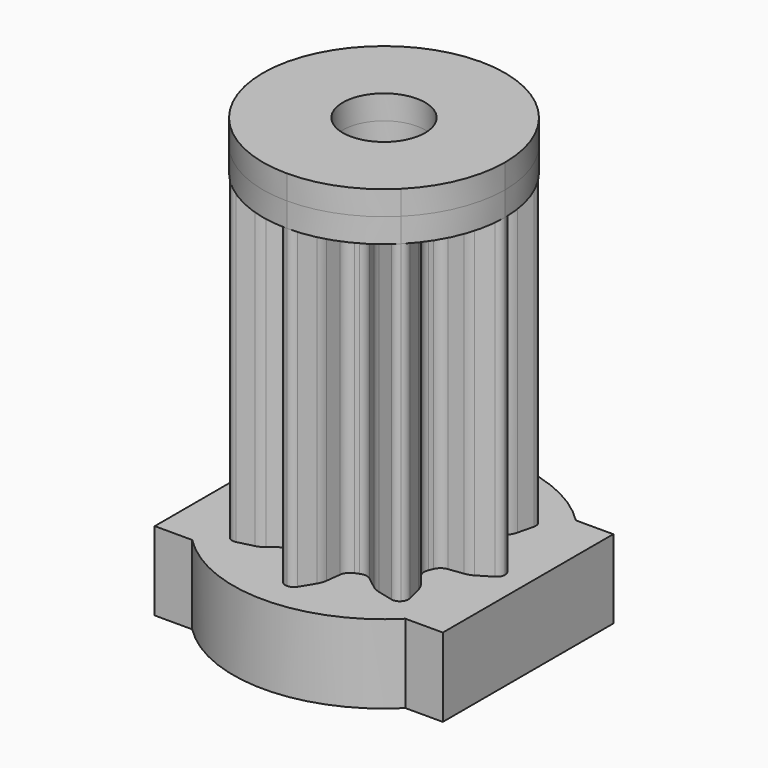
from build123d import *
from build123d import SkipClean  # not in build123d's __all__

# Parameters (mm, degrees)
F0_R     = 5
F0_R_2   = 3.15
F0_R_3   = 2.55
F1_DEPTH = 3.25
F2_R     = 2.55
F3_DEPTH = 14
F5_DEPTH = 1


# Not quite as in the source:
# - a feature names something its author has since deleted; it is built from what else it names


with BuildPart() as f1:
    # F0 (on Top) → F1 (new body)
    with BuildSketch(Plane.XY):
        with BuildLine():
            Line((-5.95, -4.4), (-4.4034787385, -4.4))
            ThreePointArc((-4.4034787385, -4.4), (0, -6.225), (4.4034787385, -4.4))
            Line((4.4034787385, -4.4), (5.95, -4.4))
            Line((5.95, -4.4), (5.95, 4.4))
            Line((5.95, 4.4), (4.4034787385, 4.4))
            ThreePointArc((4.4034787385, 4.4), (0, 6.225), (-4.4034787385, 4.4))
            Line((-4.4034787385, 4.4), (-5.95, 4.4))
            Line((-5.95, 4.4), (-5.95, -4.4))
        make_face()
        Circle(F0_R, mode=Mode.SUBTRACT)
        Circle(F0_R)
        Circle(F0_R_2, mode=Mode.SUBTRACT)
        Circle(F0_R_2)
        Circle(F0_R_3, mode=Mode.SUBTRACT)
        Circle(F0_R_3)
        with BuildLine():
            ThreePointArc((-1.275, -1.1244443072), (-0.601040764, 1.5902043894), (1.7, 0))
            ThreePointArc((1.7, 0), (1.5902043894, -0.601040764), (1.275, -1.1244443072))
            ThreePointArc((1.275, -1.1244443072), (0, -1.7), (-1.275, -1.1244443072))
        make_face(mode=Mode.SUBTRACT)
        with BuildLine():
            Line((1.275, -1.1244443072), (-1.275, -1.1244443072))
            ThreePointArc((-1.275, -1.1244443072), (0, -1.7), (1.275, -1.1244443072))
        make_face()
    extrude(amount=F1_DEPTH)

    # F2 (on face) → F3 (join)
    with BuildSketch(Plane.XY.offset(3.25)):
        with BuildLine():
            ThreePointArc((-4.8302633262, 0.3000085552), (-4.9546244936, 0.172348246), (-5, 0))
            ThreePointArc((-5, 0), (-4.9546244936, -0.172348246), (-4.8302633262, -0.3000085552))
            Line((-4.8302633262, -0.3000085552), (-4.2601369618, -0.6425750355))
            ThreePointArc((-4.2601369618, -0.6425750355), (-4.0929165173, -0.7205512094), (-3.9131380826, -0.7620563314))
            Line((-3.9131380826, -0.7620563314), (-3.3117988826, -0.835891501))
            ThreePointArc((-3.3117988826, -0.835891501), (-3.0868883315, -0.9291389359), (-2.9422567869, -1.125))
            ThreePointArc((-2.9422567869, -1.125), (-3.15, 0), (-2.9422567869, 1.125))
            ThreePointArc((-2.9422567869, 1.125), (-3.0868883315, 0.9291389359), (-3.3117988826, 0.835891501))
            Line((-3.3117988826, 0.835891501), (-3.9131380826, 0.7620563314))
            ThreePointArc((-3.9131380826, 0.7620563314), (-4.0929165173, 0.7205512094), (-4.2601369618, 0.6425750355))
            Line((-4.2601369618, 0.6425750355), (-4.8302633262, 0.3000085552))
        make_face()
        with BuildLine():
            ThreePointArc((-3.2033738691, 3.6276500367), (-3.3815799641, 3.6253171911), (-3.5355339059, 3.5355339059))
            ThreePointArc((-3.5355339059, 3.5355339059), (-3.6253171911, 3.3815799641), (-3.6276500367, 3.2033738691))
            Line((-3.6276500367, 3.2033738691), (-3.4667408995, 2.5580025694))
            ThreePointArc((-3.4667408995, 2.5580025694), (-3.4036356706, 2.3846223779), (-3.3058616735, 2.2281512744))
            Line((-3.3058616735, 2.2281512744), (-2.9328599965, 1.7507308991))
            ThreePointArc((-2.9328599965, 1.7507308991), (-2.8397601142, 1.5257592297), (-2.8759848548, 1.2849945972))
            ThreePointArc((-2.8759848548, 1.2849945972), (-2.2273863607, 2.2273863607), (-1.2849945972, 2.8759848548))
            ThreePointArc((-1.2849945972, 2.8759848548), (-1.5257592297, 2.8397601142), (-1.7507308991, 2.9328599965))
            Line((-1.7507308991, 2.9328599965), (-2.2281512744, 3.3058616735))
            ThreePointArc((-2.2281512744, 3.3058616735), (-2.3846223779, 3.4036356706), (-2.5580025694, 3.4667408995))
            Line((-2.5580025694, 3.4667408995), (-3.2033738691, 3.6276500367))
        make_face()
        with BuildLine():
            ThreePointArc((0.3000085552, 4.8302633262), (0.172348246, 4.9546244936), (0, 5))
            ThreePointArc((0, 5), (-0.172348246, 4.9546244936), (-0.3000085552, 4.8302633262))
            Line((-0.3000085552, 4.8302633262), (-0.6425750355, 4.2601369618))
            ThreePointArc((-0.6425750355, 4.2601369618), (-0.7205512094, 4.0929165173), (-0.7620563314, 3.9131380826))
            Line((-0.7620563314, 3.9131380826), (-0.835891501, 3.3117988826))
            ThreePointArc((-0.835891501, 3.3117988826), (-0.9291389359, 3.0868883315), (-1.125, 2.9422567869))
            ThreePointArc((-1.125, 2.9422567869), (0, 3.15), (1.125, 2.9422567869))
            ThreePointArc((1.125, 2.9422567869), (0.9291389359, 3.0868883315), (0.835891501, 3.3117988826))
            Line((0.835891501, 3.3117988826), (0.7620563314, 3.9131380826))
            ThreePointArc((0.7620563314, 3.9131380826), (0.7205512094, 4.0929165173), (0.6425750355, 4.2601369618))
            Line((0.6425750355, 4.2601369618), (0.3000085552, 4.8302633262))
        make_face()
        with BuildLine():
            ThreePointArc((3.2033738691, -3.6276500367), (3.3815799667, -3.6253171904), (3.5355339096, -3.5355339023))
            ThreePointArc((3.5355339096, -3.5355339023), (3.6253171918, -3.3815799616), (3.6276500367, -3.2033738691))
            Line((3.6276500367, -3.2033738691), (3.4667408995, -2.5580025694))
            ThreePointArc((3.4667408995, -2.5580025694), (3.4036356706, -2.3846223779), (3.3058616735, -2.2281512744))
            Line((3.3058616735, -2.2281512744), (2.9328599965, -1.7507308991))
            ThreePointArc((2.9328599965, -1.7507308991), (2.8397601142, -1.5257592297), (2.8759848548, -1.2849945972))
            ThreePointArc((2.8759848548, -1.2849945972), (2.2273863607, -2.2273863607), (1.2849945972, -2.8759848548))
            ThreePointArc((1.2849945972, -2.8759848548), (1.5257592297, -2.8397601142), (1.7507308991, -2.9328599965))
            Line((1.7507308991, -2.9328599965), (2.2281512744, -3.3058616735))
            ThreePointArc((2.2281512744, -3.3058616735), (2.3846223779, -3.4036356706), (2.5580025694, -3.4667408995))
            Line((2.5580025694, -3.4667408995), (3.2033738691, -3.6276500367))
        make_face()
        with BuildLine():
            ThreePointArc((-0.3000085552, -4.8302633262), (-0.172348246, -4.9546244936), (0, -5))
            ThreePointArc((0, -5), (0.172348246, -4.9546244936), (0.3000085552, -4.8302633262))
            Line((0.3000085552, -4.8302633262), (0.6425750355, -4.2601369618))
            ThreePointArc((0.6425750355, -4.2601369618), (0.7205512094, -4.0929165173), (0.7620563314, -3.9131380826))
            Line((0.7620563314, -3.9131380826), (0.835891501, -3.3117988826))
            ThreePointArc((0.835891501, -3.3117988826), (0.9291389359, -3.0868883315), (1.125, -2.9422567869))
            ThreePointArc((1.125, -2.9422567869), (0, -3.15), (-1.125, -2.9422567869))
            ThreePointArc((-1.125, -2.9422567869), (-0.9291389359, -3.0868883315), (-0.835891501, -3.3117988826))
            Line((-0.835891501, -3.3117988826), (-0.7620563314, -3.9131380826))
            ThreePointArc((-0.7620563314, -3.9131380826), (-0.7205512094, -4.0929165173), (-0.6425750355, -4.2601369618))
            Line((-0.6425750355, -4.2601369618), (-0.3000085552, -4.8302633262))
        make_face()
        with BuildLine():
            ThreePointArc((-3.6276500367, -3.2033738691), (-3.6253171911, -3.3815799641), (-3.5355339059, -3.5355339059))
            ThreePointArc((-3.5355339059, -3.5355339059), (-3.3815799641, -3.6253171911), (-3.2033738691, -3.6276500367))
            Line((-3.2033738691, -3.6276500367), (-2.5580025694, -3.4667408995))
            ThreePointArc((-2.5580025694, -3.4667408995), (-2.3846223779, -3.4036356706), (-2.2281512744, -3.3058616735))
            Line((-2.2281512744, -3.3058616735), (-1.7507308991, -2.9328599965))
            ThreePointArc((-1.7507308991, -2.9328599965), (-1.5257592297, -2.8397601142), (-1.2849945972, -2.8759848548))
            ThreePointArc((-1.2849945972, -2.8759848548), (-2.2273863607, -2.2273863607), (-2.8759848548, -1.2849945972))
            ThreePointArc((-2.8759848548, -1.2849945972), (-2.8397601142, -1.5257592297), (-2.9328599965, -1.7507308991))
            Line((-2.9328599965, -1.7507308991), (-3.3058616735, -2.2281512744))
            ThreePointArc((-3.3058616735, -2.2281512744), (-3.4036356706, -2.3846223779), (-3.4667408995, -2.5580025694))
            Line((-3.4667408995, -2.5580025694), (-3.6276500367, -3.2033738691))
        make_face()
        with BuildLine():
            ThreePointArc((2.8759848548, -1.2849945972), (2.9102205274, -1.205452812), (2.9422567869, -1.125))
            ThreePointArc((2.9422567869, -1.125), (3.0976288414, -0.5720101054), (3.15, 0))
            ThreePointArc((3.15, 0), (3.0976288414, 0.5720101054), (2.9422567869, 1.125))
            ThreePointArc((2.9422567869, 1.125), (2.9102205274, 1.205452812), (2.8759848548, 1.2849945972))
            ThreePointArc((2.8759848548, 1.2849945972), (2.2273863607, 2.2273863607), (1.2849945972, 2.8759848548))
            ThreePointArc((1.2849945972, 2.8759848548), (1.205452812, 2.9102205274), (1.125, 2.9422567869))
            ThreePointArc((1.125, 2.9422567869), (0, 3.15), (-1.125, 2.9422567869))
            ThreePointArc((-1.125, 2.9422567869), (-1.205452812, 2.9102205274), (-1.2849945972, 2.8759848548))
            ThreePointArc((-1.2849945972, 2.8759848548), (-2.2273863607, 2.2273863607), (-2.8759848548, 1.2849945972))
            ThreePointArc((-2.8759848548, 1.2849945972), (-2.9102205274, 1.205452812), (-2.9422567869, 1.125))
            ThreePointArc((-2.9422567869, 1.125), (-3.15, 0), (-2.9422567869, -1.125))
            ThreePointArc((-2.9422567869, -1.125), (-2.9102205274, -1.205452812), (-2.8759848548, -1.2849945972))
            ThreePointArc((-2.8759848548, -1.2849945972), (-2.2273863607, -2.2273863607), (-1.2849945972, -2.8759848548))
            ThreePointArc((-1.2849945972, -2.8759848548), (-1.205452812, -2.9102205274), (-1.125, -2.9422567869))
            ThreePointArc((-1.125, -2.9422567869), (0, -3.15), (1.125, -2.9422567869))
            ThreePointArc((1.125, -2.9422567869), (1.205452812, -2.9102205274), (1.2849945972, -2.8759848548))
            ThreePointArc((1.2849945972, -2.8759848548), (2.2273863607, -2.2273863607), (2.8759848548, -1.2849945972))
        make_face()
        Circle(F2_R, mode=Mode.SUBTRACT)
        Circle(F2_R)
        with BuildLine():
            Line((1.275, -1.1244443072), (-1.275, -1.1244443072))
            ThreePointArc((-1.275, -1.1244443072), (0, 1.7), (1.275, -1.1244443072))
        make_face(mode=Mode.SUBTRACT)
        with BuildLine():
            ThreePointArc((3.6276500367, 3.2033738691), (3.6253171915, 3.3815799629), (3.5355339078, 3.5355339041))
            ThreePointArc((3.5355339078, 3.5355339041), (3.3815799654, 3.6253171908), (3.2033738691, 3.6276500367))
            Line((3.2033738691, 3.6276500367), (2.5580025694, 3.4667408995))
            ThreePointArc((2.5580025694, 3.4667408995), (2.3846223779, 3.4036356706), (2.2281512744, 3.3058616735))
            Line((2.2281512744, 3.3058616735), (1.7507308991, 2.9328599965))
            ThreePointArc((1.7507308991, 2.9328599965), (1.5257592297, 2.8397601142), (1.2849945972, 2.8759848548))
            ThreePointArc((1.2849945972, 2.8759848548), (2.2273863607, 2.2273863607), (2.8759848548, 1.2849945972))
            ThreePointArc((2.8759848548, 1.2849945972), (2.8397601142, 1.5257592297), (2.9328599965, 1.7507308991))
            Line((2.9328599965, 1.7507308991), (3.3058616735, 2.2281512744))
            ThreePointArc((3.3058616735, 2.2281512744), (3.4036356706, 2.3846223779), (3.4667408995, 2.5580025694))
            Line((3.4667408995, 2.5580025694), (3.6276500367, 3.2033738691))
        make_face()
        with BuildLine():
            ThreePointArc((4.8302633262, -0.3000085552), (4.9546244936, -0.172348246), (5, 0))
            ThreePointArc((5, 0), (4.9546244936, 0.172348246), (4.8302633262, 0.3000085552))
            Line((4.8302633262, 0.3000085552), (4.2601369618, 0.6425750355))
            ThreePointArc((4.2601369618, 0.6425750355), (4.0929165173, 0.7205512094), (3.9131380826, 0.7620563314))
            Line((3.9131380826, 0.7620563314), (3.3117988826, 0.835891501))
            ThreePointArc((3.3117988826, 0.835891501), (3.0868883315, 0.9291389359), (2.9422567869, 1.125))
            ThreePointArc((2.9422567869, 1.125), (3.0976288414, 0.5720101054), (3.15, 0))
            ThreePointArc((3.15, 0), (3.0976288414, -0.5720101054), (2.9422567869, -1.125))
            ThreePointArc((2.9422567869, -1.125), (3.0868883315, -0.9291389359), (3.3117988826, -0.835891501))
            Line((3.3117988826, -0.835891501), (3.9131380826, -0.7620563314))
            ThreePointArc((3.9131380826, -0.7620563314), (4.0929165173, -0.7205512094), (4.2601369618, -0.6425750355))
            Line((4.2601369618, -0.6425750355), (4.8302633262, -0.3000085552))
        make_face()
    extrude(amount=F3_DEPTH)

    # F4 (on face) → F5 (join, symmetric)
    with BuildSketch(Plane.XY.offset(17.25)):
        with BuildLine():
            ThreePointArc((-0.3000085552, 4.8302633262), (-0.172348246, 4.9546244936), (0, 5))
            ThreePointArc((0, 5), (-1.9134171618, 4.6193976626), (-3.5355339059, 3.5355339059))
            ThreePointArc((-3.5355339059, 3.5355339059), (-3.3815799641, 3.6253171911), (-3.2033738691, 3.6276500367))
            Line((-3.2033738691, 3.6276500367), (-2.5580025694, 3.4667408995))
            ThreePointArc((-2.5580025694, 3.4667408995), (-2.3846223779, 3.4036356706), (-2.2281512744, 3.3058616735))
            Line((-2.2281512744, 3.3058616735), (-1.7507308991, 2.9328599965))
            ThreePointArc((-1.7507308991, 2.9328599965), (-1.5257592297, 2.8397601142), (-1.2849945972, 2.8759848548))
            ThreePointArc((-1.2849945972, 2.8759848548), (-1.205452812, 2.9102205274), (-1.125, 2.9422567869))
            ThreePointArc((-1.125, 2.9422567869), (-0.9291389359, 3.0868883315), (-0.835891501, 3.3117988826))
            Line((-0.835891501, 3.3117988826), (-0.7620563314, 3.9131380826))
            ThreePointArc((-0.7620563314, 3.9131380826), (-0.7205512094, 4.0929165173), (-0.6425750355, 4.2601369618))
            Line((-0.6425750355, 4.2601369618), (-0.3000085552, 4.8302633262))
        make_face()
        with BuildLine():
            ThreePointArc((-3.6276500367, 3.2033738691), (-3.6253171911, 3.3815799641), (-3.5355339059, 3.5355339059))
            ThreePointArc((-3.5355339059, 3.5355339059), (-4.6193976626, 1.9134171618), (-5, 0))
            ThreePointArc((-5, 0), (-4.9546244936, 0.172348246), (-4.8302633262, 0.3000085552))
            Line((-4.8302633262, 0.3000085552), (-4.2601369618, 0.6425750355))
            ThreePointArc((-4.2601369618, 0.6425750355), (-4.0929165173, 0.7205512094), (-3.9131380826, 0.7620563314))
            Line((-3.9131380826, 0.7620563314), (-3.3117988826, 0.835891501))
            ThreePointArc((-3.3117988826, 0.835891501), (-3.0868883315, 0.9291389359), (-2.9422567869, 1.125))
            ThreePointArc((-2.9422567869, 1.125), (-2.9102205274, 1.205452812), (-2.8759848548, 1.2849945972))
            ThreePointArc((-2.8759848548, 1.2849945972), (-2.8397601142, 1.5257592297), (-2.9328599965, 1.7507308991))
            Line((-2.9328599965, 1.7507308991), (-3.3058616735, 2.2281512744))
            ThreePointArc((-3.3058616735, 2.2281512744), (-3.4036356706, 2.3846223779), (-3.4667408995, 2.5580025694))
            Line((-3.4667408995, 2.5580025694), (-3.6276500367, 3.2033738691))
        make_face()
        with BuildLine():
            ThreePointArc((3.2033738691, 3.6276500367), (3.3815799641, 3.6253171911), (3.5355339059, 3.5355339059))
            ThreePointArc((3.5355339059, 3.5355339059), (1.9134171618, 4.6193976626), (0, 5))
            ThreePointArc((0, 5), (0.172348246, 4.9546244936), (0.3000085552, 4.8302633262))
            Line((0.3000085552, 4.8302633262), (0.6425750355, 4.2601369618))
            ThreePointArc((0.6425750355, 4.2601369618), (0.7205512094, 4.0929165173), (0.7620563314, 3.9131380826))
            Line((0.7620563314, 3.9131380826), (0.835891501, 3.3117988826))
            ThreePointArc((0.835891501, 3.3117988826), (0.9291389359, 3.0868883315), (1.125, 2.9422567869))
            ThreePointArc((1.125, 2.9422567869), (1.205452812, 2.9102205274), (1.2849945972, 2.8759848548))
            ThreePointArc((1.2849945972, 2.8759848548), (1.5257592297, 2.8397601142), (1.7507308991, 2.9328599965))
            Line((1.7507308991, 2.9328599965), (2.2281512744, 3.3058616735))
            ThreePointArc((2.2281512744, 3.3058616735), (2.3846223779, 3.4036356706), (2.5580025694, 3.4667408995))
            Line((2.5580025694, 3.4667408995), (3.2033738691, 3.6276500367))
        make_face()
        with BuildLine():
            ThreePointArc((4.8302633262, 0.3000085552), (4.9546244936, 0.172348246), (5, 0))
            ThreePointArc((5, 0), (4.6193976626, 1.9134171618), (3.5355339059, 3.5355339059))
            ThreePointArc((3.5355339059, 3.5355339059), (3.6253171911, 3.3815799641), (3.6276500367, 3.2033738691))
            Line((3.6276500367, 3.2033738691), (3.4667408995, 2.5580025694))
            ThreePointArc((3.4667408995, 2.5580025694), (3.4036356706, 2.3846223779), (3.3058616735, 2.2281512744))
            Line((3.3058616735, 2.2281512744), (2.9328599965, 1.7507308991))
            ThreePointArc((2.9328599965, 1.7507308991), (2.8397601142, 1.5257592297), (2.8759848548, 1.2849945972))
            ThreePointArc((2.8759848548, 1.2849945972), (2.9102205274, 1.205452812), (2.9422567869, 1.125))
            ThreePointArc((2.9422567869, 1.125), (3.0868883315, 0.9291389359), (3.3117988826, 0.835891501))
            Line((3.3117988826, 0.835891501), (3.9131380826, 0.7620563314))
            ThreePointArc((3.9131380826, 0.7620563314), (4.0929165173, 0.7205512094), (4.2601369618, 0.6425750355))
            Line((4.2601369618, 0.6425750355), (4.8302633262, 0.3000085552))
        make_face()
        with BuildLine():
            ThreePointArc((3.5355339059, -3.5355339059), (4.6193976626, -1.9134171618), (5, 0))
            ThreePointArc((5, 0), (4.9546244936, -0.172348246), (4.8302633262, -0.3000085552))
            Line((4.8302633262, -0.3000085552), (4.2601369618, -0.6425750355))
            ThreePointArc((4.2601369618, -0.6425750355), (4.0929165173, -0.7205512094), (3.9131380826, -0.7620563314))
            Line((3.9131380826, -0.7620563314), (3.3117988826, -0.835891501))
            ThreePointArc((3.3117988826, -0.835891501), (3.0868883315, -0.9291389359), (2.9422567869, -1.125))
            ThreePointArc((2.9422567869, -1.125), (2.9102205274, -1.205452812), (2.8759848548, -1.2849945972))
            ThreePointArc((2.8759848548, -1.2849945972), (2.8397601142, -1.5257592297), (2.9328599965, -1.7507308991))
            Line((2.9328599965, -1.7507308991), (3.3058616735, -2.2281512744))
            ThreePointArc((3.3058616735, -2.2281512744), (3.4036356706, -2.3846223779), (3.4667408995, -2.5580025694))
            Line((3.4667408995, -2.5580025694), (3.6276500367, -3.2033738691))
            ThreePointArc((3.6276500367, -3.2033738691), (3.6253171911, -3.3815799641), (3.5355339059, -3.5355339059))
        make_face()
        with BuildLine():
            ThreePointArc((0, -5), (1.9134171618, -4.6193976626), (3.5355339059, -3.5355339059))
            ThreePointArc((3.5355339059, -3.5355339059), (3.3815799641, -3.6253171911), (3.2033738691, -3.6276500367))
            Line((3.2033738691, -3.6276500367), (2.5580025694, -3.4667408995))
            ThreePointArc((2.5580025694, -3.4667408995), (2.3846223779, -3.4036356706), (2.2281512744, -3.3058616735))
            Line((2.2281512744, -3.3058616735), (1.7507308991, -2.9328599965))
            ThreePointArc((1.7507308991, -2.9328599965), (1.5257592297, -2.8397601142), (1.2849945972, -2.8759848548))
            ThreePointArc((1.2849945972, -2.8759848548), (1.205452812, -2.9102205274), (1.125, -2.9422567869))
            ThreePointArc((1.125, -2.9422567869), (0.9291389359, -3.0868883315), (0.835891501, -3.3117988826))
            Line((0.835891501, -3.3117988826), (0.7620563314, -3.9131380826))
            ThreePointArc((0.7620563314, -3.9131380826), (0.7205512094, -4.0929165173), (0.6425750355, -4.2601369618))
            Line((0.6425750355, -4.2601369618), (0.3000085552, -4.8302633262))
            ThreePointArc((0.3000085552, -4.8302633262), (0.172348246, -4.9546244936), (0, -5))
        make_face()
        with BuildLine():
            ThreePointArc((-3.5355339059, -3.5355339059), (-1.9134171618, -4.6193976626), (0, -5))
            ThreePointArc((0, -5), (-0.172348246, -4.9546244936), (-0.3000085552, -4.8302633262))
            Line((-0.3000085552, -4.8302633262), (-0.6425750355, -4.2601369618))
            ThreePointArc((-0.6425750355, -4.2601369618), (-0.7205512094, -4.0929165173), (-0.7620563314, -3.9131380826))
            Line((-0.7620563314, -3.9131380826), (-0.835891501, -3.3117988826))
            ThreePointArc((-0.835891501, -3.3117988826), (-0.9291389359, -3.0868883315), (-1.125, -2.9422567869))
            ThreePointArc((-1.125, -2.9422567869), (-1.205452812, -2.9102205274), (-1.2849945972, -2.8759848548))
            ThreePointArc((-1.2849945972, -2.8759848548), (-1.5257592297, -2.8397601142), (-1.7507308991, -2.9328599965))
            Line((-1.7507308991, -2.9328599965), (-2.2281512744, -3.3058616735))
            ThreePointArc((-2.2281512744, -3.3058616735), (-2.3846223779, -3.4036356706), (-2.5580025694, -3.4667408995))
            Line((-2.5580025694, -3.4667408995), (-3.2033738691, -3.6276500367))
            ThreePointArc((-3.2033738691, -3.6276500367), (-3.3815799641, -3.6253171911), (-3.5355339059, -3.5355339059))
        make_face()
        with BuildLine():
            ThreePointArc((-5, 0), (-4.6193976626, -1.9134171618), (-3.5355339059, -3.5355339059))
            ThreePointArc((-3.5355339059, -3.5355339059), (-3.6253171911, -3.3815799641), (-3.6276500367, -3.2033738691))
            Line((-3.6276500367, -3.2033738691), (-3.4667408995, -2.5580025694))
            ThreePointArc((-3.4667408995, -2.5580025694), (-3.4036356706, -2.3846223779), (-3.3058616735, -2.2281512744))
            Line((-3.3058616735, -2.2281512744), (-2.9328599965, -1.7507308991))
            ThreePointArc((-2.9328599965, -1.7507308991), (-2.8397601142, -1.5257592297), (-2.8759848548, -1.2849945972))
            ThreePointArc((-2.8759848548, -1.2849945972), (-2.9102205274, -1.205452812), (-2.9422567869, -1.125))
            ThreePointArc((-2.9422567869, -1.125), (-3.0868883315, -0.9291389359), (-3.3117988826, -0.835891501))
            Line((-3.3117988826, -0.835891501), (-3.9131380826, -0.7620563314))
            ThreePointArc((-3.9131380826, -0.7620563314), (-4.0929165173, -0.7205512094), (-4.2601369618, -0.6425750355))
            Line((-4.2601369618, -0.6425750355), (-4.8302633262, -0.3000085552))
            ThreePointArc((-4.8302633262, -0.3000085552), (-4.9546244936, -0.172348246), (-5, 0))
        make_face()
        with BuildLine():
            ThreePointArc((4.8302633262, -0.3000085552), (4.9546244936, -0.172348246), (5, 0))
            ThreePointArc((5, 0), (4.9546244936, 0.172348246), (4.8302633262, 0.3000085552))
            Line((4.8302633262, 0.3000085552), (4.2601369618, 0.6425750355))
            ThreePointArc((4.2601369618, 0.6425750355), (4.0929165173, 0.7205512094), (3.9131380826, 0.7620563314))
            Line((3.9131380826, 0.7620563314), (3.3117988826, 0.835891501))
            ThreePointArc((3.3117988826, 0.835891501), (3.0868883315, 0.9291389359), (2.9422567869, 1.125))
            ThreePointArc((2.9422567869, 1.125), (2.9102205274, 1.205452812), (2.8759848548, 1.2849945972))
            ThreePointArc((2.8759848548, 1.2849945972), (2.8397601142, 1.5257592297), (2.9328599965, 1.7507308991))
            Line((2.9328599965, 1.7507308991), (3.3058616735, 2.2281512744))
            ThreePointArc((3.3058616735, 2.2281512744), (3.4036356706, 2.3846223779), (3.4667408995, 2.5580025694))
            Line((3.4667408995, 2.5580025694), (3.6276500367, 3.2033738691))
            ThreePointArc((3.6276500367, 3.2033738691), (3.6253171911, 3.3815799641), (3.5355339059, 3.5355339059))
            ThreePointArc((3.5355339059, 3.5355339059), (3.3815799641, 3.6253171911), (3.2033738691, 3.6276500367))
            Line((3.2033738691, 3.6276500367), (2.5580025694, 3.4667408995))
            ThreePointArc((2.5580025694, 3.4667408995), (2.3846223779, 3.4036356706), (2.2281512744, 3.3058616735))
            Line((2.2281512744, 3.3058616735), (1.7507308991, 2.9328599965))
            ThreePointArc((1.7507308991, 2.9328599965), (1.5257592297, 2.8397601142), (1.2849945972, 2.8759848548))
            ThreePointArc((1.2849945972, 2.8759848548), (1.205452812, 2.9102205274), (1.125, 2.9422567869))
            ThreePointArc((1.125, 2.9422567869), (0.9291389359, 3.0868883315), (0.835891501, 3.3117988826))
            Line((0.835891501, 3.3117988826), (0.7620563314, 3.9131380826))
            ThreePointArc((0.7620563314, 3.9131380826), (0.7205512094, 4.0929165173), (0.6425750355, 4.2601369618))
            Line((0.6425750355, 4.2601369618), (0.3000085552, 4.8302633262))
            ThreePointArc((0.3000085552, 4.8302633262), (0.172348246, 4.9546244936), (0, 5))
            ThreePointArc((0, 5), (-0.172348246, 4.9546244936), (-0.3000085552, 4.8302633262))
            Line((-0.3000085552, 4.8302633262), (-0.6425750355, 4.2601369618))
            ThreePointArc((-0.6425750355, 4.2601369618), (-0.7205512094, 4.0929165173), (-0.7620563314, 3.9131380826))
            Line((-0.7620563314, 3.9131380826), (-0.835891501, 3.3117988826))
            ThreePointArc((-0.835891501, 3.3117988826), (-0.9291389359, 3.0868883315), (-1.125, 2.9422567869))
            ThreePointArc((-1.125, 2.9422567869), (-1.205452812, 2.9102205274), (-1.2849945972, 2.8759848548))
            ThreePointArc((-1.2849945972, 2.8759848548), (-1.5257592297, 2.8397601142), (-1.7507308991, 2.9328599965))
            Line((-1.7507308991, 2.9328599965), (-2.2281512744, 3.3058616735))
            ThreePointArc((-2.2281512744, 3.3058616735), (-2.3846223779, 3.4036356706), (-2.5580025694, 3.4667408995))
            Line((-2.5580025694, 3.4667408995), (-3.2033738691, 3.6276500367))
            ThreePointArc((-3.2033738691, 3.6276500367), (-3.3815799641, 3.6253171911), (-3.5355339059, 3.5355339059))
            ThreePointArc((-3.5355339059, 3.5355339059), (-3.6253171911, 3.3815799641), (-3.6276500367, 3.2033738691))
            Line((-3.6276500367, 3.2033738691), (-3.4667408995, 2.5580025694))
            ThreePointArc((-3.4667408995, 2.5580025694), (-3.4036356706, 2.3846223779), (-3.3058616735, 2.2281512744))
            Line((-3.3058616735, 2.2281512744), (-2.9328599965, 1.7507308991))
            ThreePointArc((-2.9328599965, 1.7507308991), (-2.8397601142, 1.5257592297), (-2.8759848548, 1.2849945972))
            ThreePointArc((-2.8759848548, 1.2849945972), (-2.9102205274, 1.205452812), (-2.9422567869, 1.125))
            ThreePointArc((-2.9422567869, 1.125), (-3.0868883315, 0.9291389359), (-3.3117988826, 0.835891501))
            Line((-3.3117988826, 0.835891501), (-3.9131380826, 0.7620563314))
            ThreePointArc((-3.9131380826, 0.7620563314), (-4.0929165173, 0.7205512094), (-4.2601369618, 0.6425750355))
            Line((-4.2601369618, 0.6425750355), (-4.8302633262, 0.3000085552))
            ThreePointArc((-4.8302633262, 0.3000085552), (-4.9546244936, 0.172348246), (-5, 0))
            ThreePointArc((-5, 0), (-4.9546244936, -0.172348246), (-4.8302633262, -0.3000085552))
            Line((-4.8302633262, -0.3000085552), (-4.2601369618, -0.6425750355))
            ThreePointArc((-4.2601369618, -0.6425750355), (-4.0929165173, -0.7205512094), (-3.9131380826, -0.7620563314))
            Line((-3.9131380826, -0.7620563314), (-3.3117988826, -0.835891501))
            ThreePointArc((-3.3117988826, -0.835891501), (-3.0868883315, -0.9291389359), (-2.9422567869, -1.125))
            ThreePointArc((-2.9422567869, -1.125), (-2.9102205274, -1.205452812), (-2.8759848548, -1.2849945972))
            ThreePointArc((-2.8759848548, -1.2849945972), (-2.8397601142, -1.5257592297), (-2.9328599965, -1.7507308991))
            Line((-2.9328599965, -1.7507308991), (-3.3058616735, -2.2281512744))
            ThreePointArc((-3.3058616735, -2.2281512744), (-3.4036356706, -2.3846223779), (-3.4667408995, -2.5580025694))
            Line((-3.4667408995, -2.5580025694), (-3.6276500367, -3.2033738691))
            ThreePointArc((-3.6276500367, -3.2033738691), (-3.6253171911, -3.3815799641), (-3.5355339059, -3.5355339059))
            ThreePointArc((-3.5355339059, -3.5355339059), (-3.3815799641, -3.6253171911), (-3.2033738691, -3.6276500367))
            Line((-3.2033738691, -3.6276500367), (-2.5580025694, -3.4667408995))
            ThreePointArc((-2.5580025694, -3.4667408995), (-2.3846223779, -3.4036356706), (-2.2281512744, -3.3058616735))
            Line((-2.2281512744, -3.3058616735), (-1.7507308991, -2.9328599965))
            ThreePointArc((-1.7507308991, -2.9328599965), (-1.5257592297, -2.8397601142), (-1.2849945972, -2.8759848548))
            ThreePointArc((-1.2849945972, -2.8759848548), (-1.205452812, -2.9102205274), (-1.125, -2.9422567869))
            ThreePointArc((-1.125, -2.9422567869), (-0.9291389359, -3.0868883315), (-0.835891501, -3.3117988826))
            Line((-0.835891501, -3.3117988826), (-0.7620563314, -3.9131380826))
            ThreePointArc((-0.7620563314, -3.9131380826), (-0.7205512094, -4.0929165173), (-0.6425750355, -4.2601369618))
            Line((-0.6425750355, -4.2601369618), (-0.3000085552, -4.8302633262))
            ThreePointArc((-0.3000085552, -4.8302633262), (-0.172348246, -4.9546244936), (0, -5))
            ThreePointArc((0, -5), (0.172348246, -4.9546244936), (0.3000085552, -4.8302633262))
            Line((0.3000085552, -4.8302633262), (0.6425750355, -4.2601369618))
            ThreePointArc((0.6425750355, -4.2601369618), (0.7205512094, -4.0929165173), (0.7620563314, -3.9131380826))
            Line((0.7620563314, -3.9131380826), (0.835891501, -3.3117988826))
            ThreePointArc((0.835891501, -3.3117988826), (0.9291389359, -3.0868883315), (1.125, -2.9422567869))
            ThreePointArc((1.125, -2.9422567869), (1.205452812, -2.9102205274), (1.2849945972, -2.8759848548))
            ThreePointArc((1.2849945972, -2.8759848548), (1.5257592297, -2.8397601142), (1.7507308991, -2.9328599965))
            Line((1.7507308991, -2.9328599965), (2.2281512744, -3.3058616735))
            ThreePointArc((2.2281512744, -3.3058616735), (2.3846223779, -3.4036356706), (2.5580025694, -3.4667408995))
            Line((2.5580025694, -3.4667408995), (3.2033738691, -3.6276500367))
            ThreePointArc((3.2033738691, -3.6276500367), (3.3815799641, -3.6253171911), (3.5355339059, -3.5355339059))
            ThreePointArc((3.5355339059, -3.5355339059), (3.6253171911, -3.3815799641), (3.6276500367, -3.2033738691))
            Line((3.6276500367, -3.2033738691), (3.4667408995, -2.5580025694))
            ThreePointArc((3.4667408995, -2.5580025694), (3.4036356706, -2.3846223779), (3.3058616735, -2.2281512744))
            Line((3.3058616735, -2.2281512744), (2.9328599965, -1.7507308991))
            ThreePointArc((2.9328599965, -1.7507308991), (2.8397601142, -1.5257592297), (2.8759848548, -1.2849945972))
            ThreePointArc((2.8759848548, -1.2849945972), (2.9102205274, -1.205452812), (2.9422567869, -1.125))
            ThreePointArc((2.9422567869, -1.125), (3.0868883315, -0.9291389359), (3.3117988826, -0.835891501))
            Line((3.3117988826, -0.835891501), (3.9131380826, -0.7620563314))
            ThreePointArc((3.9131380826, -0.7620563314), (4.0929165173, -0.7205512094), (4.2601369618, -0.6425750355))
            Line((4.2601369618, -0.6425750355), (4.8302633262, -0.3000085552))
        make_face()
        with BuildLine():
            ThreePointArc((-1.275, -1.1244443072), (-0.601040764, 1.5902043894), (1.7, 0))
            ThreePointArc((1.7, 0), (1.5902043894, -0.601040764), (1.275, -1.1244443072))
            ThreePointArc((1.275, -1.1244443072), (0, -1.7), (-1.275, -1.1244443072))
        make_face(mode=Mode.SUBTRACT)
    with SkipClean():  # cleaning this boolean's faces spoils the solid; the shape is the same uncleaned
        extrude(amount=F5_DEPTH, both=True)


solid = f1.part
